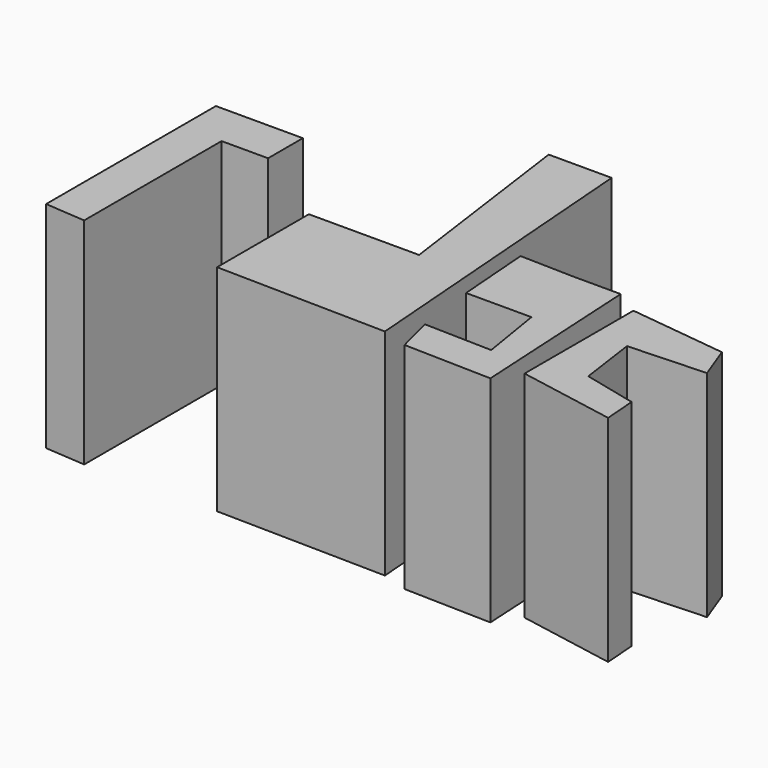
from build123d import *

# Parameters (mm, degrees)
F1_DEPTH = 25.4


# Not quite as in the source:
# - a feature of the source that left no trace in its solid (it failed there, or was rolled back) is left out


with BuildPart() as f1:
    # F0 (on Top) → F1 (new body)
    with BuildSketch(Plane.XY):
        Polygon((-58.8288158178, 20.6982176751), (-69.1107288003, 20.6982176751), (-69.1107288003, -4.3861074373), (-64.3243193626, -4.7406563535), (-64.3243193626, 15.5572602525), (-58.8288158178, 15.5572602525), align=None)
    extrude(amount=F1_DEPTH)


with BuildPart() as f1b:
    # F0 (on Top) → F1, piece 2 (new body)
    with BuildSketch(Plane.XY):
        Polygon((-35.8717851341, 9.1753825545), (-41.1013774574, 9.1753825545), (-48.9014498889, 9.1753825545), (-48.9014498889, -4.3861074373), (-28.7808086723, -4.7406563535), (-31.6171981394, 32.3096886277), (-39.0627235174, 32.3096886277), align=None)
    extrude(amount=F1_DEPTH)


with BuildPart() as f1c:
    # F0 (on Top) → F1, piece 3 (new body)
    with BuildSketch(Plane.XY):
        Polygon((-16.4547897875, 14.6912075579), (-22.0323093235, 14.6912075579), (-28.418160975, 14.8528749123), (-27.7362425849, 5.9453141228), (-20.0114697218, 5.9453141228), (-18.7959093807, -1.5165152081), (-26.8014892936, -1.3138420181), (-25.6768274582, -5.7131264287), (-15.3231201693, -5.9752459638), align=None)
    extrude(amount=F1_DEPTH)


with BuildPart() as f1d:
    # F0 (on Top) → F1, piece 4 (new body)
    with BuildSketch(Plane.XY):
        Polygon((-8.5331005976, 0), (-9.5031037927, 6.9311829284), (-0.3689071746, 7.3353513144), (-1.9047448877, 11.4578641951), (-13.463947922, 12.8320353106), (-13.463947922, -3.2538492233), (-1.9047448877, -5.3555215709), (-2.1986400516, -1.5165152081), align=None)
    extrude(amount=F1_DEPTH)


solid = Compound([f1.part, f1b.part, f1c.part, f1d.part])
